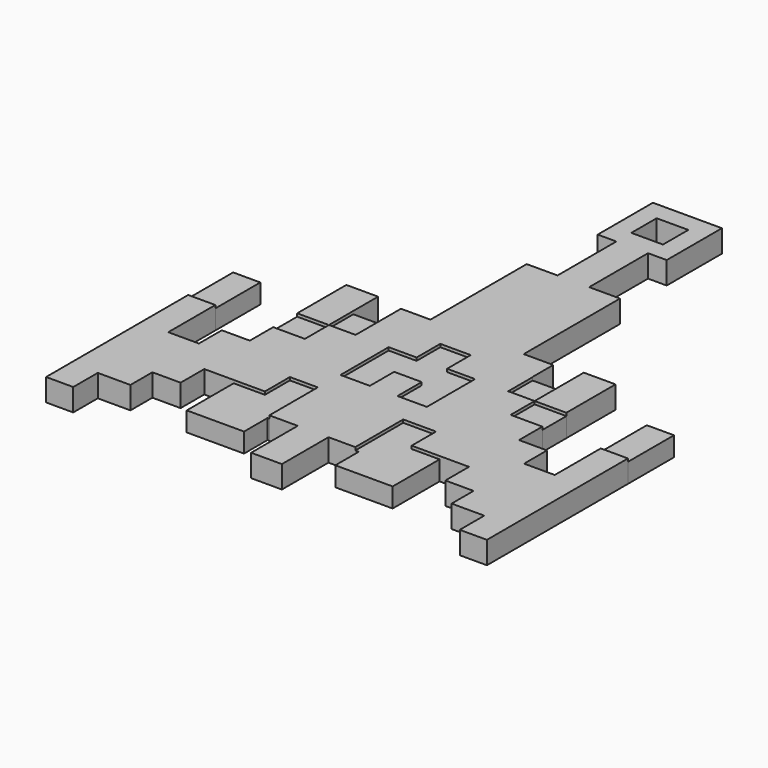
from build123d import *

# Parameters (mm, degrees)
F1_DEPTH = 3
F0_W     = 3.6364123225
F0_H     = 7.5237620622
F2_DEPTH = 2.6
F0_W_2   = 3.5404209048
F0_H_2   = 4.0894895792
F0_H_3   = 7.7040316537
F0_W_3   = 4.2472146451
F0_H_4   = 4.0195640177
F0_W_4   = 3.5795867443


# Not quite as in the source:
# - a feature names something its author has since deleted; it is built from what else it names


with BuildPart() as f1:
    # F0 (on Top) → F1 (new body)
    with BuildSketch(Plane.XY):
        Polygon((32.3127042502, 67.4153068662), (30.1925335079, 67.4153068662), (28.0723627657, 67.4153068662), (28.0723627657, 64.9153068662), (28.0723627657, 55.0648160279), (23.9476244897, 55.0648160279), (23.9476244897, 38.9564856887), (19.9987087399, 38.9564856887), (19.9987087399, 35.4621224105), (19.9987087399, 31.3726328313), (16.4191219956, 31.3726328313), (16.4191219956, 27.3530688137), (12.1719073504, 27.3530688137), (12.1719073504, 23.4449207783), (8.4218550473, 23.4449207783), (8.4218550473, 19.6096431464), (4.3172221631, 19.6096431464), (4.3172221631, 27.4939443916), (0.6808098406, 27.4939443916), (0.6808098406, 3.7104797084), (4.3172221631, 3.7104797084), (4.3172221631, 7.8136157244), (8.6926203221, 7.8136157244), (8.6926203221, 11.48981601), (12.4692637473, 11.48981601), (12.4692637473, 15.447255224), (16.406616196, 15.447255224), (20.5889474601, 15.447255224), (20.5889474601, 19.6236893535), (24.331657216, 19.6236893535), (24.331657216, 11.5099046379), (28.1328521669, 11.5099046379), (28.1328521669, 3.7104797084), (29.953636229, 3.7104797084), (30.4314307868, 3.7104797084), (32.252214849, 3.7104797084), (32.252214849, 11.5099046379), (35.8404926956, 11.5099046379), (35.8404926956, 19.530121237), (40.2381792665, 19.530121237), (40.2381792665, 15.447255224), (43.9784508198, 15.447255224), (47.9158032686, 15.447255224), (47.9158032686, 11.48981601), (51.6924466938, 11.48981601), (51.6924466938, 7.8136157244), (56.0678448528, 7.8136157244), (56.0678448528, 3.7104797084), (59.7042571753, 3.7104797084), (59.7042571753, 27.3136748001), (56.0678448528, 27.3136748001), (56.0678448528, 19.6096431464), (51.9632119685, 19.6096431464), (51.9632119685, 23.4449207783), (48.2131596655, 23.4449207783), (48.2131596655, 27.3530688137), (44.0051108599, 27.3530688137), (43.9659450203, 27.3530688137), (43.9659450203, 31.3726328313), (40.4255241156, 31.3726328313), (40.4255241156, 35.4621224105), (40.386358276, 35.4621224105), (40.386358276, 38.9564856887), (36.4374425262, 38.9564856887), (36.4374425262, 55.0648160279), (32.3127042502, 55.0648160279), (32.3127042502, 64.9153068662), align=None)
        Polygon((28.1724799424, 31.3594639301), (28.1724799424, 35.3187546134), (32.251752913, 35.3187546134), (32.251752913, 31.3594639301), (35.9961111099, 31.3594639301), (35.9961111099, 23.2938230038), (32.0594422519, 23.2938230038), (32.0594422519, 27.3549240083), (28.3647906035, 27.3549240083), (28.3647906035, 23.2938230038), (24.4281217456, 23.2938230038), (24.4281217456, 31.3594639301), align=None, mode=Mode.SUBTRACT)
        Polygon((32.3127042502, 71.6556483507), (32.3127042502, 67.4153068662), (32.3127042502, 64.9153068662), (34.8127042502, 64.9153068662), (34.8127042502, 74.1556483507), (25.5723627657, 74.1556483507), (25.5723627657, 64.9153068662), (28.0723627657, 64.9153068662), (28.0723627657, 67.4153068662), (28.0723627657, 71.6556483507), align=None)
    extrude(amount=F1_DEPTH)


with BuildPart() as f1b:
    # F0 (on Top) → F1, piece 2 (new body)
    with BuildSketch(Plane.XY):
        Polygon((43.9659450203, 39.5989455283), (43.9659450203, 35.4621224105), (43.9659450203, 31.3726328313), (44.0051108599, 31.3726328313), (48.2131596655, 31.3726328313), (48.2131596655, 39.5989455283), (44.0051108599, 39.5989455283), align=None)
    extrude(amount=F1_DEPTH)


with BuildPart() as f1c:
    # F0 (on Top) → F1, piece 3 (new body)
    with BuildSketch(Plane.XY):
        Polygon((16.4191219956, 31.3726328313), (16.4191219956, 35.4621224105), (16.4191219956, 39.5989455283), (12.1719073504, 39.5989455283), (12.1719073504, 31.3726328313), align=None)
    extrude(amount=F1_DEPTH)


with BuildPart() as f2:
    # F0 (on Top) → F2 (new body)
    with BuildSketch(Plane.XY):
        with Locations((2.4990160018, 31.2558254227)):
            Rectangle(F0_W, F0_H)
    extrude(amount=F2_DEPTH)


with BuildPart() as f2b:
    # F0 (on Top) → F2, piece 2 (new body)
    with BuildSketch(Plane.XY):
        Polygon((32.251752913, 35.3187546134), (28.1724799424, 35.3187546134), (28.1724799424, 31.3594639301), (24.4281217456, 31.3594639301), (24.4281217456, 23.2938230038), (28.3647906035, 23.2938230038), (28.3647906035, 27.3549240083), (32.0594422519, 27.3549240083), (32.0594422519, 23.2938230038), (35.9961111099, 23.2938230038), (35.9961111099, 31.3594639301), (32.251752913, 31.3594639301), align=None)
    extrude(amount=F2_DEPTH)


with BuildPart() as f2c:
    # F0 (on Top) → F2, piece 3 (new body)
    with BuildSketch(Plane.XY):
        with Locations((42.1957345679, 33.4173776209)):
            Rectangle(F0_W_2, F0_H_2)
    extrude(amount=F2_DEPTH)


with BuildPart() as f2d:
    # F0 (on Top) → F2, piece 4 (new body)
    with BuildSketch(Plane.XY):
        with Locations((57.8860510141, 31.1656906269)):
            Rectangle(F0_W, F0_H_3)
    extrude(amount=F2_DEPTH)


with BuildPart() as f2e:
    # F0 (on Top) → F2, piece 5 (new body)
    with BuildSketch(Plane.XY):
        Polygon((43.9784508198, 7.5926417485), (43.9784508198, 15.447255224), (40.2381792665, 15.447255224), (40.2381792665, 19.530121237), (35.8404926956, 19.530121237), (35.8404926956, 11.5099046379), (36.3046396524, 11.5099046379), (36.3046396524, 7.5926417485), align=None)
    extrude(amount=F2_DEPTH)


with BuildPart() as f2f:
    # F0 (on Top) → F2, piece 6 (new body)
    with BuildSketch(Plane.XY):
        Polygon((20.5889474601, 15.447255224), (16.406616196, 15.447255224), (16.406616196, 7.5926417485), (24.0804273635, 7.5926417485), (24.0804273635, 11.5099046379), (24.331657216, 11.5099046379), (24.331657216, 19.6236893535), (20.5889474601, 19.6236893535), align=None)
    extrude(amount=F2_DEPTH)


with BuildPart() as f2g:
    # F0 (on Top) → F2, piece 7 (new body)
    with BuildSketch(Plane.XY):
        with Locations((14.295514673, 29.3628508225)):
            Rectangle(F0_W_3, F0_H_4)
    extrude(amount=F2_DEPTH)


with BuildPart() as f2h:
    # F0 (on Top) → F2, piece 8 (new body)
    with BuildSketch(Plane.XY):
        with Locations((18.2089153677, 33.4173776209)):
            Rectangle(F0_W_4, F0_H_2)
    extrude(amount=F2_DEPTH)


with BuildPart() as f2i:
    # F0 (on Top) → F2, piece 9 (new body)
    with BuildSketch(Plane.XY):
        Polygon((44.0051108599, 31.3726328313), (43.9659450203, 31.3726328313), (43.9659450203, 27.3530688137), (44.0051108599, 27.3530688137), (48.2131596655, 27.3530688137), (48.2131596655, 31.3726328313), align=None)
    extrude(amount=F2_DEPTH)


solid = Compound([f1.part, f1b.part, f1c.part, f2.part, f2b.part, f2c.part, f2d.part, f2e.part, f2f.part, f2g.part, f2h.part, f2i.part])
